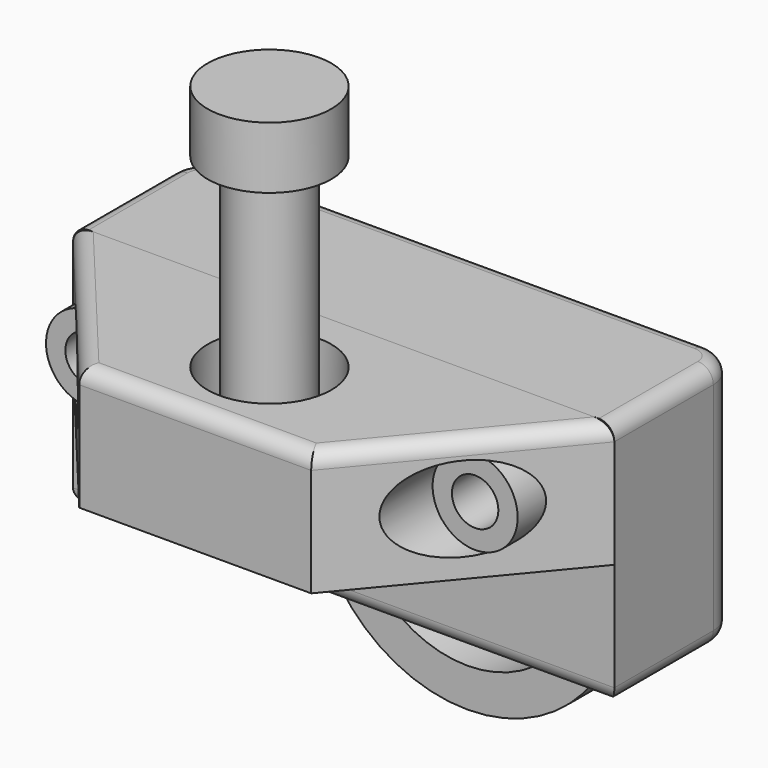
from build123d import *

# Parameters (mm, degrees)
F0_R      = 4
F1_DEPTH  = 8
F0_R_2    = 2.5
F2_DEPTH  = 4
F3_DEPTH  = 20
F4_R      = 4
F5_DEPTH  = 4
F6_R      = 1.5
F7_DEPTH  = 12.001
F6_R_2    = 2.75
F8_DEPTH  = 5
F9_R      = 2.75
F10_DEPTH = 7.001
F11_R     = 1
F12_DEPTH = 8
F13_R     = 1.5
F14_DEPTH = 22.001
F15_DEPTH = 5
F16_R     = 1
F17_E39_W = 2.5
F17_E39_H = 2


with BuildPart() as f1:
    # F0 (on Top) → F1 (new body)
    with BuildSketch(Plane.XY):
        Polygon((-10, 12), (0, 0), (15, 0), (25, 12), (15, 12), (0, 12), align=None)
        with Locations((7.5, 6)):
            Circle(F0_R, mode=Mode.SUBTRACT)
    extrude(amount=F1_DEPTH)

    # F0 (on Top) → F2 (join)
    with BuildSketch(Plane.XY):
        with Locations((7.5, 6)):
            Circle(F0_R)
        with Locations((7.5, 6)):
            Circle(F0_R_2, mode=Mode.SUBTRACT)
    extrude(amount=F2_DEPTH)

    # F6 (on face) → F7 (cut, through all)
    with BuildSketch(Plane(origin=(0, 12, 0), x_dir=(-1, 0, 0), z_dir=(0, 1, 0))):
        with Locations((-20, 4)):
            Circle(F6_R)
        with Locations((5, 4)):
            Circle(F6_R)
    extrude(amount=-F7_DEPTH, mode=Mode.SUBTRACT)

    # F6 (on face) → F8 (join)
    with BuildSketch(Plane(origin=(0, 12, 0), x_dir=(-1, 0, 0), z_dir=(0, 1, 0))):
        with Locations((-20, 4)):
            Circle(F6_R_2)
        with Locations((-20, 4)):
            Circle(F6_R, mode=Mode.SUBTRACT)
        with Locations((5, 4)):
            Circle(F6_R_2)
        with Locations((5, 4)):
            Circle(F6_R, mode=Mode.SUBTRACT)
    extrude(amount=-F8_DEPTH)

    # F9 (on face) → F10 (cut, through all)
    with BuildSketch(Plane.XZ.offset(-7)):
        with Locations((20, 4)):
            Circle(F9_R)
        with Locations((-5, 4)):
            Circle(F9_R)
    extrude(amount=F10_DEPTH, mode=Mode.SUBTRACT)

    # F11
    f11_edges = [f1.edges().sort_by_distance(p)[0] for p in [
        (-5, 6, 8),
        (7.5, 0, 8),
        (20, 6, 8),
    ]]
    fillet(f11_edges, radius=F11_R)


with BuildPart() as f3:
    # F0 (on Top) → F3 (new body)
    with BuildSketch(Plane.XY):
        with Locations((7.5, 6)):
            Circle(F0_R_2)
    extrude(amount=F3_DEPTH)

    # F4 (on face) → F5 (join)
    with BuildSketch(Plane.XY.offset(20)):
        with Locations((7.5, 6)):
            Circle(F4_R)
    extrude(amount=F5_DEPTH)


with BuildPart() as f12:
    # F0 (on Top) → F12 (new body, symmetric)
    with BuildSketch(Plane.XY):
        with BuildLine():
            Line((-10, 20), (-10, 12))
            Line((-10, 12), (0, 12))
            Line((0, 12), (15, 12))
            Line((15, 12), (25, 12))
            Line((25, 12), (25, 20))
            ThreePointArc((25, 20), (24.4142135624, 21.4142135624), (23, 22))
            Line((23, 22), (-8, 22))
            ThreePointArc((-8, 22), (-9.4142135624, 21.4142135624), (-10, 20))
        make_face()
    extrude(amount=F12_DEPTH, both=True)

    # F13 (on face) → F14 (cut, through all)
    with BuildSketch(Plane(origin=(0, 22, 0), x_dir=(-1, 0, 0), z_dir=(0, 1, 0))):
        with Locations((-20, 4)):
            Circle(F13_R)
        with Locations((5, 4)):
            Circle(F13_R)
    extrude(amount=-F14_DEPTH, mode=Mode.SUBTRACT)

    # F13 (on face) → F15 (cut)
    with BuildSketch(Plane(origin=(0, 22, 0), x_dir=(-1, 0, 0), z_dir=(0, 1, 0))):
        with Locations((-10, 4.3301270189)):
            Circle(F13_R)
        with Locations((-12.5, 0)):
            Circle(F13_R)
        with Locations((-5, 4.3301270189)):
            Circle(F13_R)
        with Locations((-10, -4.3301270189)):
            Circle(F13_R)
        with Locations((-5, -4.3301270189)):
            Circle(F13_R)
        with Locations((-2.5, 0)):
            Circle(F13_R)
    extrude(amount=-F15_DEPTH, mode=Mode.SUBTRACT)

    # F16
    f16_edges = [f12.edges().sort_by_distance(p)[0] for p in [
        (25, 16, 8),
        (25, 16, -8),
        (7.5, 12, -8),
    ]]
    fillet(f16_edges, radius=F16_R)


with BuildPart() as f18:
    # F18: sweep along a path in F13
    with BuildLine(Plane(origin=(0, 22, 0), x_dir=(-1, 0, 0), z_dir=(0, 1, 0))) as f18_path:
        Line((-16.25, 1), (-16.25, -8))
        ThreePointArc((-16.25, -8), (-7.5, -16.75), (1.25, -8))
        Line((1.25, -8), (1.25, 1))
    # F17_E39 (on explicit) → F18 (sweep)
    with BuildSketch(Plane(origin=(15, 22, 1), x_dir=(1, 0, 0), z_dir=(0, 0, 1))):
        with Locations((1.25, 1)):
            Rectangle(F17_E39_W, F17_E39_H)
    sweep(path=f18_path.line)


solid = Compound([f1.part, f3.part, f12.part, f18.part])
